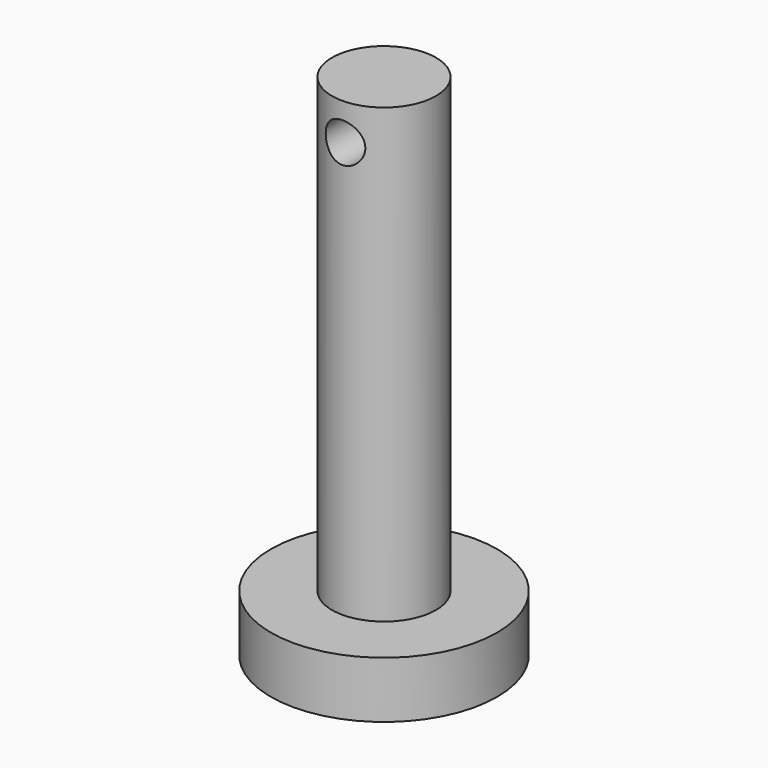
from build123d import *

# Parameters (mm, degrees)
F0_R     = 2.335
F1_DEPTH = 20.32
F2_R     = 5.08
F2_R_2   = 2.335
F3_DEPTH = 2.54
F4_R     = 0.889
F5_DEPTH = 12.7


with BuildPart() as f1:
    # F0 (on Top) → F1 (new body)
    with BuildSketch(Plane.XY):
        Circle(F0_R)
    extrude(amount=F1_DEPTH)

    # F2 (on face) → F3 (join)
    with BuildSketch(Plane(origin=(0, 0, 0), x_dir=(1, 0, 0), z_dir=(0, 0, -1))):
        Circle(F2_R)
        Circle(F2_R_2, mode=Mode.SUBTRACT)
        Circle(F2_R_2)
    extrude(amount=F3_DEPTH)

    # F4 (on Front) → F5 (cut, symmetric)
    with BuildSketch(Plane.XZ):
        with Locations((0, 18.669)):
            Circle(F4_R)
    extrude(amount=F5_DEPTH, both=True, mode=Mode.SUBTRACT)


solid = f1.part
